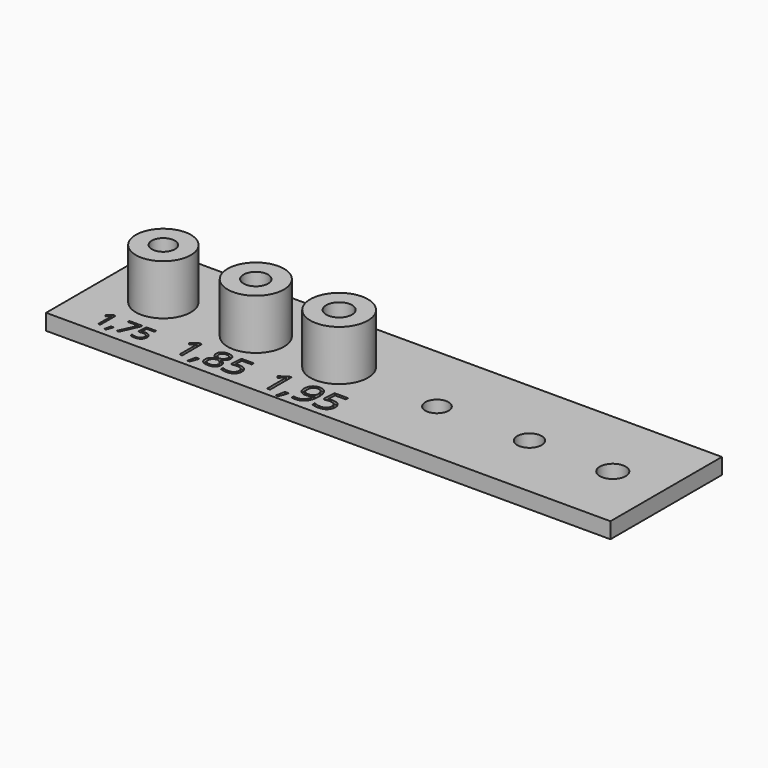
from build123d import *

# Parameters (mm, degrees)
F0_W           = 42.5833122038
F0_H           = 10.513080284
F1_DEPTH       = 5
F2_R           = 0.875
F2_R_2         = 0.925
F2_R_3         = 0.975
F3_DEPTH       = 25
F4_T           = -1.2
F5_R           = 0.875
F5_R_2         = 0.925
F5_R_3         = 0.975
F6_DEPTH       = 25
F8_START       = 1
F7_TEXT_SIZE   = 2.0343279983
F7_TEXT_SIZE_2 = 2.6000327327
F7_TEXT_SIZE_3 = 2.8357353887
F8_DEPTH       = 0.5


# Not quite as in the source:
# - Text() gives the source's letters only with a copy of the font that has no kerning and outlines rounded to 1/6400 em; it was checked with that copy


with BuildPart() as f1:
    # F0 (on Top) → F1 (new body)
    with BuildSketch(Plane.XY):
        with Locations((-54.3839537155, 15.0026036426)):
            Rectangle(F0_W, F0_H)
    extrude(amount=F1_DEPTH)

    # F2 (on face) → F3 (cut)
    with BuildSketch(Plane.XY.offset(5)):
        with Locations((-71.1254999042, 15.1182382833)):
            Circle(F2_R)
        with Locations((-64.1495361924, 15.1182382833)):
            Circle(F2_R_2)
        with Locations((-57.8618049622, 15.1182382833)):
            Circle(F2_R_3)
    extrude(amount=-F3_DEPTH, mode=Mode.SUBTRACT)

    # F4
    f4_openings = [f1.faces().sort_by_distance(p)[0] for p in [
        (-54.209012, 15.000478, 5),
        (-54.383954, 9.746064, 2.5),
        (-33.092298, 15.002604, 2.5),
        (-54.383954, 20.259144, 2.5),
        (-75.67561, 15.002604, 2.5),
    ]]
    offset(amount=F4_T, openings=f4_openings)

    # F5 (on Top) → F6 (cut)
    with BuildSketch(Plane.XY):
        with Locations((-50.2255000174, 14.8013444268)):
            Circle(F5_R)
        with Locations((-43.2495363057, 14.8013444268)):
            Circle(F5_R_2)
        with Locations((-36.9618050754, 14.8013444268)):
            Circle(F5_R_3)
    extrude(amount=F6_DEPTH, mode=Mode.SUBTRACT)

    # F7 (on Top) → F8 (cut)
    with BuildSketch(Plane.XY.offset(F8_START)):
        with Locations((-72.9383602738, 10.5405524373)):
            Text('1,75', F7_TEXT_SIZE, font='Open Sans', text_align=(TextAlign.LEFT, TextAlign.BOTTOM))
        with Locations((-136.5541219711, 23.0306647718)):
            Text('1,75', F7_TEXT_SIZE, font='Open Sans', text_align=(TextAlign.LEFT, TextAlign.BOTTOM))
        with Locations((-141.0942226648, 21.5223450214)):
            Text('1,75', F7_TEXT_SIZE, font='Open Sans', text_align=(TextAlign.LEFT, TextAlign.BOTTOM))
        with Locations((-203.7651389837, 33.9166689664)):
            Text('1,75', F7_TEXT_SIZE, font='Open Sans', text_align=(TextAlign.LEFT, TextAlign.BOTTOM))
        with Locations((-66.9146776199, 10.5009833351)):
            Text('1,85', F7_TEXT_SIZE_2, font='Open Sans', text_align=(TextAlign.LEFT, TextAlign.BOTTOM))
        with Locations((-60.2288374126, 10.3312774227)):
            Text('1,95', F7_TEXT_SIZE_3, font='Open Sans', text_align=(TextAlign.LEFT, TextAlign.BOTTOM))
    extrude(amount=F8_DEPTH, mode=Mode.SUBTRACT)


solid = f1.part
